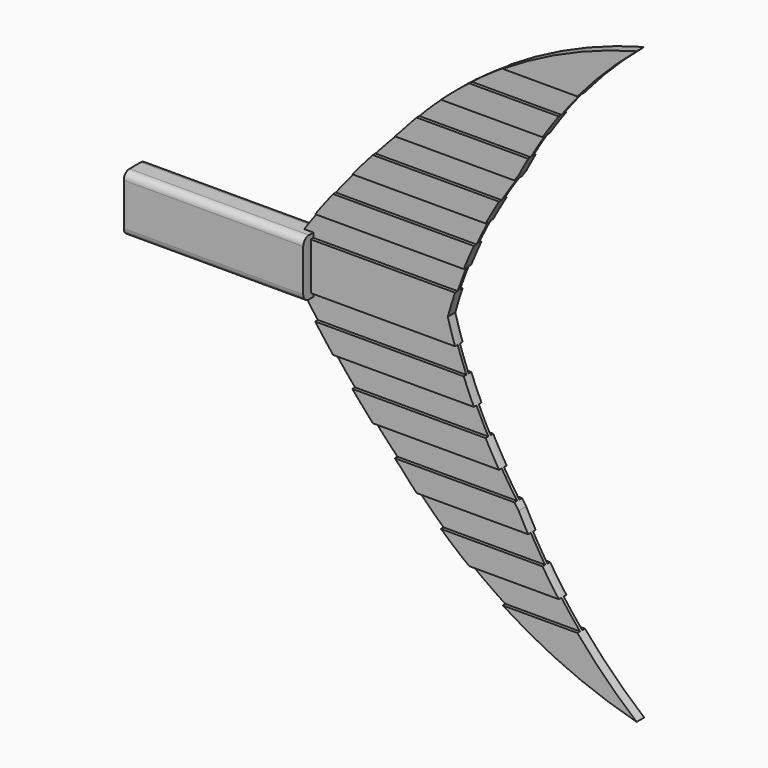
from build123d import *

# Parameters (mm, degrees)
F1_DEPTH         = 1
F4_DEPTH         = 0.7
F4_COPIES2_COUNT = 2
F5_W             = 38
F5_H             = 12
F6_DEPTH         = 3
F7_R             = 1.5


# Not quite as in the source:
# - a pattern or mirror of a feature is missing from the dataset's text; its kind, count and spacing are read off the source's solid


with BuildPart() as f1:
    # F0 (on Front) → F1 (new body, symmetric)
    with BuildSketch(Plane.XZ):
        with BuildLine():
            ThreePointArc((25, 31.25), (11.7164027855, 16.2518777716), (0, 0))
            Line((0, 0), (35, 0))
            ThreePointArc((35, 0), (41.1356304071, 16.2798974046), (50, 31.25))
            Line((50, 31.25), (25, 31.25))
        make_face()
        with BuildLine():
            ThreePointArc((75, 62.5), (47.6444357815, 50.6439027497), (25, 31.25))
            Line((25, 31.25), (50, 31.25))
            ThreePointArc((50, 31.25), (60.9207680237, 48.138385581), (75, 62.5))
        make_face()
    extrude(amount=F1_DEPTH, both=True)

    # F2: F1 across plane


with BuildPart() as f1_1:
    add(f1.part)
    add(f1.part.mirror(Plane.XY))

    # F3 (on face) → F4 (cut)
    with BuildSketch(Plane.XZ.offset(1)):
        with BuildLine():
            Line((38.3820565676, 10), (6.9138783475, 10))
            ThreePointArc((6.9138783475, 10), (5.1100506614, 7.5137050995), (3.3446205931, 5))
            Line((3.3446205931, 5), (36.543888556, 5))
            ThreePointArc((36.543888556, 5), (37.4296717705, 7.5122424899), (38.3820565676, 10))
        make_face()
        with BuildLine():
            ThreePointArc((14.7901250767, 20), (12.736458423, 17.5163842045), (10.7230770186, 15))
            Line((10.7230770186, 15), (40.5323833312, 15))
            ThreePointArc((40.5323833312, 15), (41.7401268698, 17.5173495329), (43.0176791325, 20))
            Line((43.0176791325, 20), (14.7901250767, 20))
        make_face()
        with BuildLine():
            ThreePointArc((23.7864537922, 30), (21.4399722373, 27.5198472862), (19.1361704174, 25))
            Line((19.1361704174, 25), (45.8671764928, 25))
            ThreePointArc((45.8671764928, 25), (47.4556813757, 27.5242471055), (49.1187564845, 30))
            Line((49.1187564845, 30), (23.7864537922, 30))
        make_face()
        with BuildLine():
            ThreePointArc((33.5555945556, 40), (30.9391304542, 37.5461308043), (28.4123585311, 35))
            Line((28.4123585311, 35), (52.0223589414, 35))
            ThreePointArc((52.0223589414, 35), (53.5018795741, 37.5221680923), (55.0545103176, 40))
            Line((55.0545103176, 40), (33.5555945556, 40))
        make_face()
        with BuildLine():
            ThreePointArc((46.6278522844, 50), (43.0272085219, 47.5769747675), (39.5350905643, 45))
            Line((39.5350905643, 45), (58.5103303946, 45))
            ThreePointArc((58.5103303946, 45), (60.4389654659, 47.5313247859), (62.4471689161, 50))
            Line((62.4471689161, 50), (46.6278522844, 50))
        make_face()
    f4 = extrude(amount=-F4_DEPTH, mode=Mode.SUBTRACT)

    # F4_copies: F4 across plane
    add(f4.mirror(Plane.ZX), mode=Mode.SUBTRACT)

    # F4_copies1: F4 across plane
    add(f4.mirror(Plane(origin=(0, 0, 0), x_dir=(-1, 0, 0), z_dir=(0, 0, -1))), mode=Mode.SUBTRACT)

    # F4_copies2: F4 ×2 about axis
    f4_copies2_axis = Axis((0, 0, 0), (1, 0, 0))
    for i in range(1, F4_COPIES2_COUNT):
        add(f4.rotate(f4_copies2_axis, i * 360 / F4_COPIES2_COUNT), mode=Mode.SUBTRACT)

    # F5 (on Front) → F6 (join, symmetric)
    with BuildSketch(Plane.XZ):
        with Locations((-13, 0)):
            Rectangle(F5_W, F5_H)
    extrude(amount=F6_DEPTH, both=True)

    # F7
    f7_edges = [f1_1.edges().sort_by_distance(p)[0] for p in [
        (-13, 3, 6),
        (-13, -3, 6),
        (-13, -3, -6),
        (-13, 3, -6),
    ]]
    fillet(f7_edges, radius=F7_R)


solid = f1_1.part
